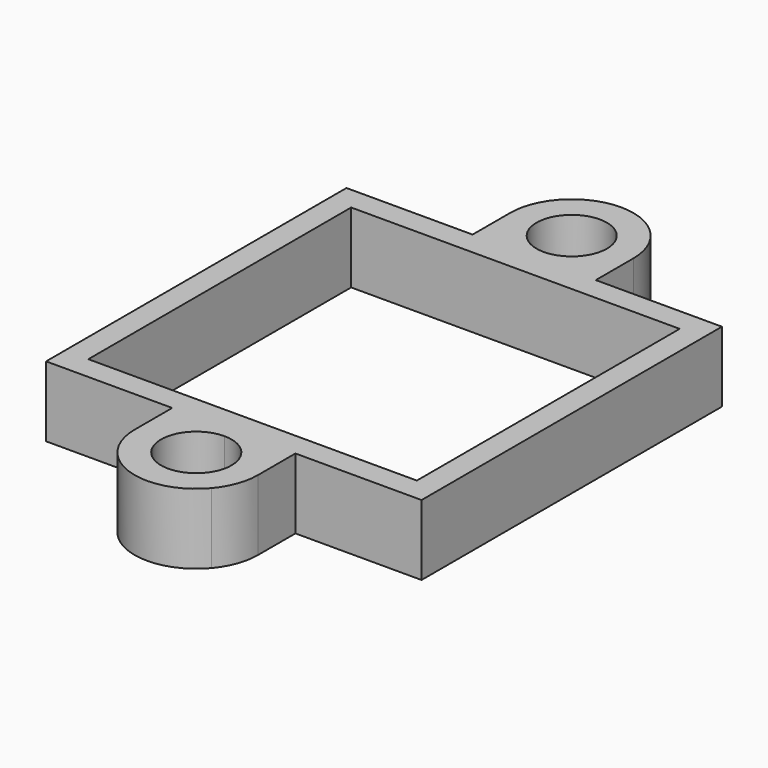
from build123d import *

# Parameters (mm, degrees)
F0_W     = 14
F0_H     = 14
F1_DEPTH = 3


# Not quite as in the source:
# - a feature names something its author has since deleted; it is built from what else it names


with BuildPart() as f1:
    # F0 (on Top) → F1 (new body)
    with BuildSketch(Plane.XY):
        with BuildLine():
            Line((2.625, -8), (8, -8))
            Line((8, -8), (8, 8))
            Line((8, 8), (2.625, 8))
            Line((2.625, 8), (2, 8))
            Line((2, 8), (1.7001838136, 8))
            ThreePointArc((1.7001838136, 8), (0, 7.375), (-1.7001838136, 8))
            Line((-1.7001838136, 8), (-2, 8))
            Line((-2, 8), (-2.625, 8))
            Line((-2.625, 8), (-8, 8))
            Line((-8, 8), (-8, -8))
            Line((-8, -8), (-2.625, -8))
            Line((-2.625, -8), (-2, -8))
            Line((-2, -8), (-1.7001838136, -8))
            ThreePointArc((-1.7001838136, -8), (0, -7.375), (1.7001838136, -8))
            Line((1.7001838136, -8), (2, -8))
            Line((2, -8), (2.625, -8))
        make_face()
        Rectangle(F0_W, F0_H, mode=Mode.SUBTRACT)
        with BuildLine():
            Line((2.625, -10), (2.625, -8))
            Line((2.625, -8), (2, -8))
            Line((2, -8), (2, -8.2998161864))
            ThreePointArc((2, -8.2998161864), (2.4638004181, -9.0942889534), (2.625, -10))
        make_face()
        with BuildLine():
            Line((2, -8.2998161864), (2, -8))
            Line((2, -8), (1.7001838136, -8))
            ThreePointArc((1.7001838136, -8), (1.8561553006, -8.1438446994), (2, -8.2998161864))
        make_face()
        with BuildLine():
            ThreePointArc((2, -11.7001838136), (2.4638004181, -10.9057110466), (2.625, -10))
            ThreePointArc((2.625, -10), (2.4638004181, -9.0942889534), (2, -8.2998161864))
            Line((2, -8.2998161864), (2, -11.7001838136))
        make_face()
        with BuildLine():
            Line((2, 8), (2.625, 8))
            Line((2.625, 8), (2.625, 10))
            ThreePointArc((2.625, 10), (2.382604406, 8.8982644398), (1.7001838136, 8))
            Line((1.7001838136, 8), (2, 8))
        make_face()
        with BuildLine():
            ThreePointArc((2, -8.2998161864), (1.8561553006, -8.1438446994), (1.7001838136, -8))
            Line((1.7001838136, -8), (0, -8))
            Line((0, -8), (-1.7001838136, -8))
            ThreePointArc((-1.7001838136, -8), (-2.382604406, -8.8982644398), (-2.625, -10))
            ThreePointArc((-2.625, -10), (-0.9057110466, -12.4638004181), (2, -11.7001838136))
            Line((2, -11.7001838136), (2, -8.2998161864))
        make_face()
        with BuildLine():
            ThreePointArc((1.5, -10), (-1.0606601718, -11.0606601718), (0, -8.5))
            ThreePointArc((0, -8.5), (1.0606601718, -8.9393398282), (1.5, -10))
        make_face(mode=Mode.SUBTRACT)
        with BuildLine():
            Line((0, -8), (1.7001838136, -8))
            ThreePointArc((1.7001838136, -8), (0, -7.375), (-1.7001838136, -8))
            Line((-1.7001838136, -8), (0, -8))
        make_face()
        with BuildLine():
            ThreePointArc((1.7001838136, 8), (2.382604406, 8.8982644398), (2.625, 10))
            ThreePointArc((2.625, 10), (0, 12.625), (-2.625, 10))
            ThreePointArc((-2.625, 10), (-2.382604406, 8.8982644398), (-1.7001838136, 8))
            Line((-1.7001838136, 8), (0, 8))
            Line((0, 8), (1.7001838136, 8))
        make_face()
        with BuildLine():
            ThreePointArc((1.5, 10), (1.0606601718, 8.9393398282), (0, 8.5))
            ThreePointArc((0, 8.5), (-1.0606601718, 11.0606601718), (1.5, 10))
        make_face(mode=Mode.SUBTRACT)
        with BuildLine():
            ThreePointArc((-2.625, -10), (-2.382604406, -8.8982644398), (-1.7001838136, -8))
            Line((-1.7001838136, -8), (-2, -8))
            Line((-2, -8), (-2.625, -8))
            Line((-2.625, -8), (-2.625, -10))
        make_face()
        with BuildLine():
            ThreePointArc((-1.7001838136, 8), (0, 7.375), (1.7001838136, 8))
            Line((1.7001838136, 8), (0, 8))
            Line((0, 8), (-1.7001838136, 8))
        make_face()
        with BuildLine():
            ThreePointArc((-1.7001838136, 8), (-2.382604406, 8.8982644398), (-2.625, 10))
            Line((-2.625, 10), (-2.625, 8))
            Line((-2.625, 8), (-2, 8))
            Line((-2, 8), (-1.7001838136, 8))
        make_face()
    extrude(amount=F1_DEPTH)


solid = f1.part
